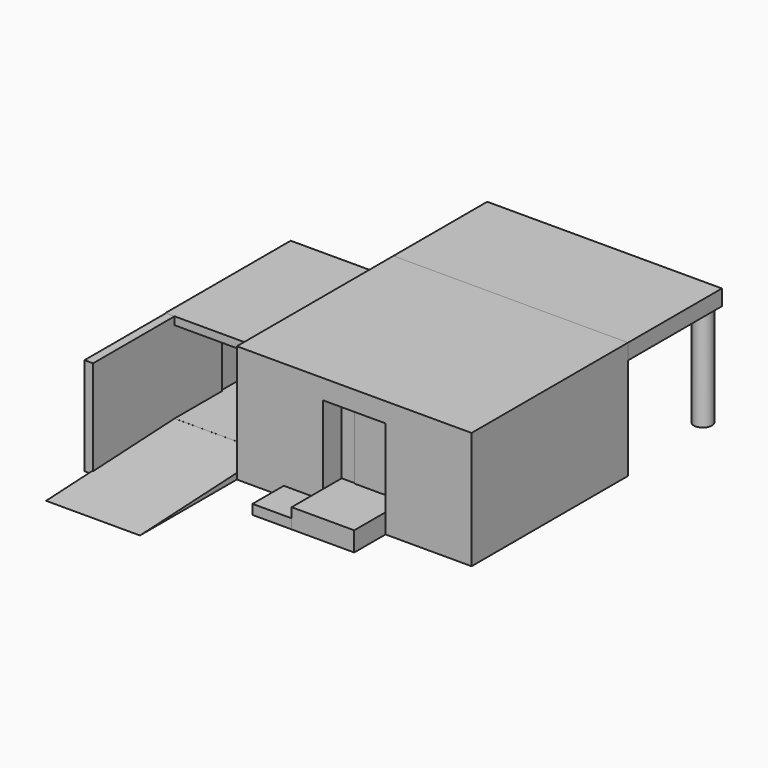
from build123d import *

# Parameters (mm, degrees)
F1_DEPTH  = 38.1
F2_W      = 76.2
F2_H      = 5.08
F3_DEPTH  = 38.1
F5_W      = 20.32
F5_H      = 6.35
F6_DEPTH  = 7.62
F8_W      = 2.794
F8_H      = 31.75
F9_DEPTH  = 52.324
F10_DEPTH = 20.32
F11_W     = 12.7857104659
F11_H     = 3.175
F12_DEPTH = 12.7
F13_W     = 5.791861964
F13_H     = 20.9366468877
F14_DEPTH = 0.254
F15_W     = 33.02
F15_H     = 50.8
F16_DEPTH = 31.75
F17_DEPTH = 30.48
F18_T     = -2.54
F19_R     = 2.9147550464
F20_DEPTH = 33.02


with BuildPart() as f1:
    # F0 (on Top) → F1 (new body)
    with BuildSketch(Plane.XY):
        Polygon((-38.1, -31.75), (-10.16, -31.75), (-10.16, -24.13), (10.16, -24.13), (10.16, -31.75), (38.1, -31.75), (38.1, 31.75), (-38.1, 31.75), (-38.1, -19.05), align=None)
    extrude(amount=F1_DEPTH)

    # F5 (on face) → F6 (join)
    with BuildSketch(Plane.XZ.offset(24.13)):
        with Locations((0, 34.925)):
            Rectangle(F5_W, F5_H)
    extrude(amount=F6_DEPTH)


with BuildPart() as f3:
    # F2 (on face) → F3 (new body)
    with BuildSketch(Plane(origin=(0, 31.75, 0), x_dir=(-1, 0, 0), z_dir=(0, 1, 0))):
        with Locations((0, 35.56)):
            Rectangle(F2_W, F2_H)
    extrude(amount=F3_DEPTH)


with BuildPart() as f9:
    # F8 (on Front) → F9 (new body)
    with BuildSketch(Plane.XZ):
        with Locations((-69.723, 15.875)):
            Rectangle(F8_W, F8_H)
    extrude(amount=F9_DEPTH)


with BuildPart() as f10:
    # F5 (on face) → F10 (new body)
    with BuildSketch(Plane.XZ.offset(24.13)):
        with Locations((0, 3.175)):
            Rectangle(F5_W, F5_H)
    extrude(amount=F10_DEPTH)


with BuildPart() as f12:
    # F11 (on face) → F12 (new body)
    with BuildSketch(Plane(origin=(-10.16, 0, 0), x_dir=(0, -1, 0), z_dir=(-1, 0, 0))):
        with Locations((38.057144767, 1.5875)):
            Rectangle(F11_W, F11_H)
    extrude(amount=F12_DEPTH)


with BuildPart() as f14:
    # F13 (on face) → F14 (new body)
    with BuildSketch(Plane.XZ.offset(24.13)):
        with Locations((2.895930982, 16.8183234438)):
            Rectangle(F13_W, F13_H)
        with Locations((-2.895930982, 16.8183234438)):
            Rectangle(F13_W, F13_H)
    extrude(amount=F14_DEPTH)


with BuildPart() as f16:
    # F15 (on Top) → F16 (new body)
    with BuildSketch(Plane.XY):
        with Locations((-54.7516793013, 6.1444475591)):
            Rectangle(F15_W, F15_H)
    extrude(amount=F16_DEPTH)

    # F18
    f18_openings = [f16.faces().sort_by_distance(p)[0] for p in [
        (-54.751679, -19.255552, 15.875),
    ]]
    offset(amount=F18_T, openings=f18_openings)


with BuildPart() as f17:
    # F7 (on face) → F17 (new body)
    with BuildSketch(Plane(origin=(-38.1, 0, 0), x_dir=(0, -1, 0), z_dir=(-1, 0, 0))):
        Polygon((31.75, 1.9199459951), (19.05, 2.54), (19.05, 0), (31.75, 0), align=None)
        Polygon((71.07450068, 0), (31.75, 1.9199459951), (31.75, 0), align=None)
    extrude(amount=F17_DEPTH)


with BuildPart() as f20:
    # F19 (on face) → F20 (new body)
    with BuildSketch(Plane(origin=(0, 0, 33.02), x_dir=(1, 0, 0), z_dir=(0, 0, -1))):
        with Locations((34.5117524266, -66.6021332145)):
            Circle(F19_R)
    extrude(amount=F20_DEPTH)


with BuildPart() as f20b:
    # F19 (on face) → F20, piece 2 (new body)
    with BuildSketch(Plane(origin=(0, 0, 33.02), x_dir=(1, 0, 0), z_dir=(0, 0, -1))):
        with Locations((-34.5117524266, -66.6021332145)):
            Circle(F19_R)
    extrude(amount=F20_DEPTH)


solid = Compound([f1.part, f3.part, f9.part, f10.part, f12.part, f14.part, f16.part, f17.part, f20.part, f20b.part])
